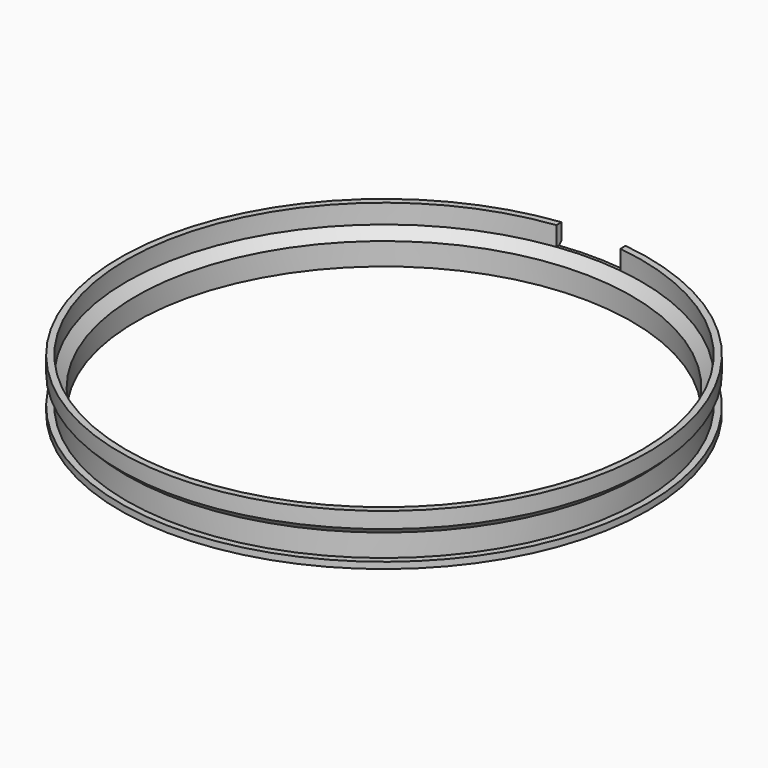
from build123d import *

# Parameters (mm, degrees)
F0_R          = 41.25
F0_R_2        = 40.25
F1_DEPTH      = 3
F1_DEPTH_BACK = 1
F0_R_3        = 38.75
F2_DEPTH      = 5
F3_S5_R       = 40.25
F3_T6_DEPTH   = 60
F3_S11_R      = 40.25
F3_T12_DEPTH  = 58
F4_R          = 41.25
F4_R_2        = 40.25
F5_DEPTH      = 1
F7_END_RADIUS = 41.25
F6_W          = 10
F6_H          = 3
F7_REACH      = 51.6913065089


# Not quite as in the source:
# - a fillet or chamfer that OpenCascade refuses, or shapes differently, is made with other operations: its cross-section is extruded or revolved along the edge and cut away or added


with BuildPart() as f1:
    # F0 (on Top) → F1 (new body, two sides)
    with BuildSketch(Plane.XY) as f1_sk:
        Circle(F0_R)
        Circle(F0_R_2, mode=Mode.SUBTRACT)
    extrude(amount=F1_DEPTH)
    extrude(f1_sk.sketch, amount=-F1_DEPTH_BACK)

    # F0 (on Top) → F2 (join)
    with BuildSketch(Plane.XY):
        Circle(F0_R_2)
        Circle(F0_R_3, mode=Mode.SUBTRACT)
    extrude(amount=-F2_DEPTH)

    # F3: chamfer of 1.5 on 2 edges, made by hand


with BuildPart() as f3_tool2:
    # F3_s3 → F3_t4 (revolve)
    with BuildSketch(Plane.XZ):
        Polygon((41.25, 0.5), (39.75, -1), (41.25, -1), align=None)
    revolve(axis=Axis((0, 0, -1), (0, 0, 1)))

    # F3_s5 → F3_t6 (cut, symmetric)
    with BuildSketch(Plane.XY.offset(-0.3)):
        Circle(F3_S5_R)
    extrude(amount=F3_T6_DEPTH, both=True, mode=Mode.SUBTRACT)


with BuildPart() as f1_1:
    add(f1.part)

    # F3_t1: cut F3_tool2
    add(f3_tool2.part, mode=Mode.SUBTRACT)


with BuildPart() as f3_tool8:
    # F3_s9 → F3_t10 (revolve)
    with BuildSketch(Plane.XZ):
        Polygon((40.25, 0), (38.75, -1.5), (38.75, 0), align=None)
    revolve(axis=Axis((0, 0, 0), (0, 0, 1)))

    # F3_s11 → F3_t12 (intersect, symmetric)
    with BuildSketch(Plane.XY.offset(-0.8)):
        Circle(F3_S11_R)
    extrude(amount=F3_T12_DEPTH, both=True, mode=Mode.INTERSECT)


with BuildPart() as f1_2:
    add(f1_1.part)

    # F3_t7: cut F3_tool8
    add(f3_tool8.part, mode=Mode.SUBTRACT)

    # F4 (on face) → F5 (join)
    with BuildSketch(Plane(origin=(0, 0, -5), x_dir=(1, 0, 0), z_dir=(0, 0, -1))):
        Circle(F4_R)
        Circle(F4_R_2, mode=Mode.SUBTRACT)
    extrude(amount=-F5_DEPTH)

    f7_end = (Plane(origin=(0, 0, 1.75), x_dir=(-1, 0, 0), z_dir=(0, 0, -1)) * Cylinder(F7_END_RADIUS, 337.2757510104, mode=Mode.PRIVATE)).faces().sort_by_distance((-41.25, 0, 1.75))[0]
    # F6 (on Front) → F7 (cut, up to the whole of a round face its end follows)
    with BuildSketch(Plane.XZ):
        with Locations((0, 1.5)):
            Rectangle(F6_W, F6_H)
    f7_long = extrude(amount=-F7_REACH, mode=Mode.PRIVATE)
    add(split(f7_long, bisect_by=f7_end, keep=Keep.BOTTOM, mode=Mode.PRIVATE), mode=Mode.SUBTRACT)


solid = f1_2.part
